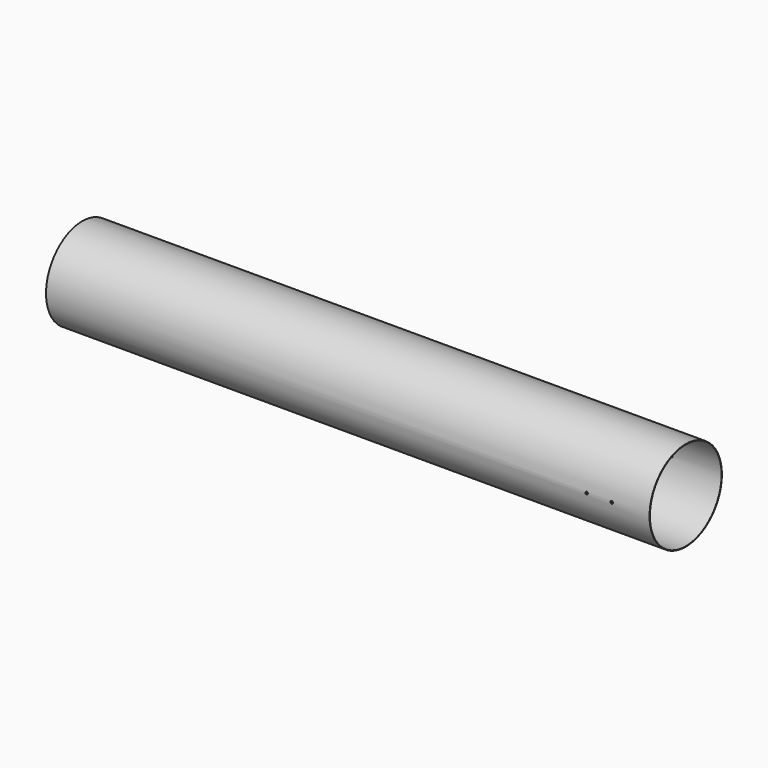
from build123d import *

# Parameters (mm, degrees)
F0_R     = 457.2
F0_R_2   = 452.4375
F1_DEPTH = 6096
F3_DEPTH = 1216.152
F4_DEPTH = 466.598


# Not quite as in the source:
# - a pattern or mirror of a feature is missing from the dataset's text; its kind, count and spacing are read off the source's solid


with BuildPart() as f1:
    # F0 (on Right) → F1 (new body)
    with BuildSketch(Plane.YZ):
        Circle(F0_R)
        Circle(F0_R_2, mode=Mode.SUBTRACT)
    extrude(amount=F1_DEPTH)

    # F2 (on Front) → F3 (cut)
    with BuildSketch(Plane.XZ):
        with BuildLine():
            ThreePointArc((5727.7, 0), (5715, 12.7), (5702.3, 0))
            ThreePointArc((5702.3, 0), (5715, -12.7), (5727.7, 0))
        make_face()
    f3 = extrude(amount=F3_DEPTH, mode=Mode.SUBTRACT)

    # F3_copies: F3 across plane
    add(f3.mirror(Plane(origin=(5587.999873, 0.001565, 8e-06), x_dir=(0, 0, -1), z_dir=(-1, 0, 0))), mode=Mode.SUBTRACT)

    # F2 (on Front) → F4 (cut)
    with BuildSketch(Plane.XZ):
        with BuildLine():
            Line((5588, 0), (5575.3, 0))
            ThreePointArc((5575.3, 0), (5588, -12.7), (5600.7, 0))
            Line((5600.7, 0), (5588, 0))
        make_face()
        with BuildLine():
            ThreePointArc((5600.7, 0), (5588, 12.7), (5575.3, 0))
            Line((5575.3, 0), (5588, 0))
            Line((5588, 0), (5600.7, 0))
        make_face()
    extrude(amount=-F4_DEPTH, mode=Mode.SUBTRACT)


solid = f1.part
